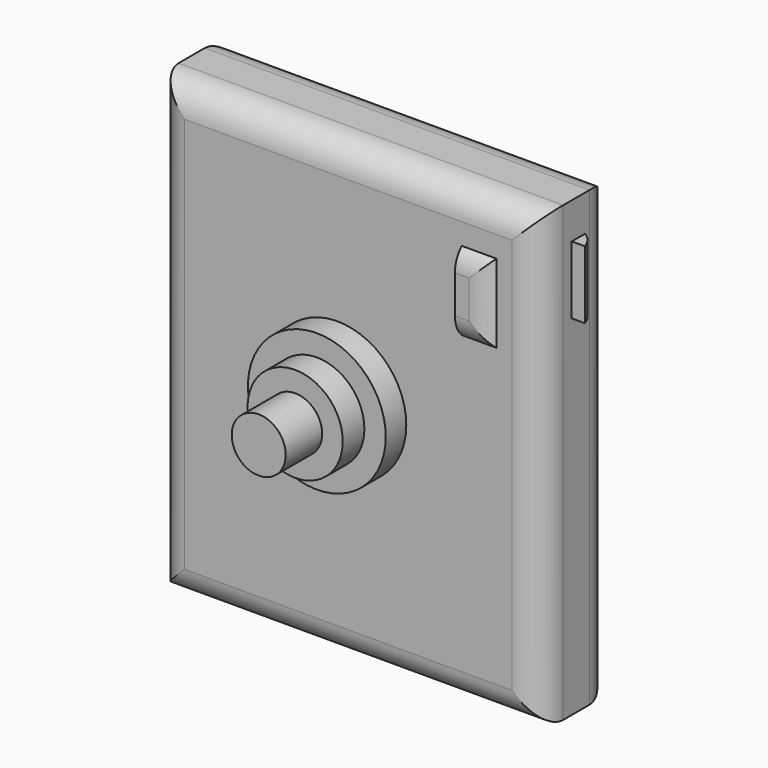
from build123d import *

# Parameters (mm, degrees)
F0_W         = 68.5527212918
F0_H         = 80.7738155127
F1_DEPTH     = 16.002
F2_R         = 12.2829248395
F2_W         = 6.1860904098
F2_H         = 13.9971412718
F4_DEPTH     = 1.524
F5_DEPTH     = 3.048
F3_W         = 2.9572332278
F3_H         = 12.0760332793
F6_DEPTH     = 2.54
F7_T1_DEPTH  = 34.0730785354
F8_R         = 8.4752207388
F9_DEPTH     = 4.826
F10_R        = 4.8104699567
F11_DEPTH    = 8.128
F12_R        = 5.08
F13_T1_DEPTH = 32.1363694803
F13_T3_DEPTH = 24.3253186183
F14_W        = 41.5736716241
F14_H        = 57.9494982958
F15_DEPTH    = 1.016


# Not quite as in the source:
# - a fillet or chamfer that OpenCascade refuses, or shapes differently, is made with other operations: its cross-section is extruded or revolved along the edge and cut away or added


with BuildPart() as f1:
    # F0 (on Front) → F1 (new body)
    with BuildSketch(Plane.XZ):
        with Locations((1.9095446914, -0.1909546554)):
            Rectangle(F0_W, F0_H)
    extrude(amount=F1_DEPTH)

    # F2 (on face) → F4 (join)
    with BuildSketch(Plane.XZ.offset(16.002)):
        Circle(F2_R)
        with Locations((25.2598635852, 24.3296492845)):
            Rectangle(F2_W, F2_H)
    extrude(amount=F4_DEPTH)

    # F5 (add): a face of the model
    f5_faces = [f1.faces().sort_by_distance(p)[0] for p in [
        (0, -17.526, 0),
    ]]
    extrude(f5_faces, amount=F5_DEPTH)

    # F3 (on face) → F6 (join)
    with BuildSketch(Plane.YZ.offset(36.1859053373)):
        with Locations((-7.535086479, 27.7017401531)):
            Rectangle(F3_W, F3_H)
    extrude(amount=F6_DEPTH)

    # F7: fillet of radius 5.08 on 1 edges, made by hand

    # F7_s2 → F7_t1 (cut)
    with BuildSketch(Plane.XY.offset(10.6652008854)):
        with BuildLine():
            ThreePointArc((36.1859053373, -6.0564698651), (38.0453143886, -7.9158789164), (38.7259053373, -10.4558789164))
            Line((38.7259053373, -10.4558789164), (38.7259053373, -6.0564698651))
            Line((38.7259053373, -6.0564698651), (36.1859053373, -6.0564698651))
        make_face()
    extrude(amount=F7_T1_DEPTH, mode=Mode.SUBTRACT)

    # F8 (on face) → F9 (join)
    with BuildSketch(Plane.XZ.offset(20.574)):
        Circle(F8_R)
    extrude(amount=F9_DEPTH)

    # F10 (on face) → F11 (join)
    with BuildSketch(Plane.XZ.offset(25.4)):
        Circle(F10_R)
    extrude(amount=F11_DEPTH)

    # F12
    f12_edges = [f1.edges().sort_by_distance(p)[0] for p in [
        (36.185905, -16.002, -0.190955),
        (1.909545, -16.002, 40.195953),
        (1.909545, -16.002, -40.577862),
        (-32.366816, -16.002, -0.190955),
        (1.909545, 0, -40.577862),
        (36.185905, 0, -0.190955),
        (1.909545, 0, 40.195953),
        (-32.366816, 0, -0.190955),
    ]]
    fillet(f12_edges, radius=F12_R)

    # F13: fillet of radius 5.08 on 3 edges, made by hand

    # F13_s2 → F13_t1 (cut)
    with BuildSketch(Plane.XY.offset(8.2614645443)):
        with BuildLine():
            ThreePointArc((28.3529087901, -16.002), (26.6925386883, -17.1295285843), (24.7250631484, -17.526))
            Line((24.7250631484, -17.526), (28.3529087901, -17.526))
            Line((28.3529087901, -17.526), (28.3529087901, -16.002))
        make_face()
    extrude(amount=F13_T1_DEPTH, mode=Mode.SUBTRACT)

    # F13_s4 → F13_t3 (cut)
    with BuildSketch(Plane.YZ.offset(13.0972042761)):
        with BuildLine():
            ThreePointArc((-16.002, 31.3282199204), (-17.1295285843, 29.6678498186), (-17.526, 27.7003742787))
            Line((-17.526, 27.7003742787), (-17.526, 31.3282199204))
            Line((-17.526, 31.3282199204), (-16.002, 31.3282199204))
        make_face()
        with BuildLine():
            ThreePointArc((-16.002, 17.3310786486), (-17.1295285843, 18.9914487504), (-17.526, 20.9589242903))
            Line((-17.526, 20.9589242903), (-17.526, 17.3310786486))
            Line((-17.526, 17.3310786486), (-16.002, 17.3310786486))
        make_face()
    extrude(amount=F13_T3_DEPTH, mode=Mode.SUBTRACT)

    # F14 (on face) → F15 (join)
    with BuildSketch(Plane(origin=(0, 0, 0), x_dir=(-1, 0, 0), z_dir=(0, 1, 0))):
        with Locations((-1.9210586324, 0.1702420413)):
            Rectangle(F14_W, F14_H)
    extrude(amount=F15_DEPTH)


solid = f1.part
